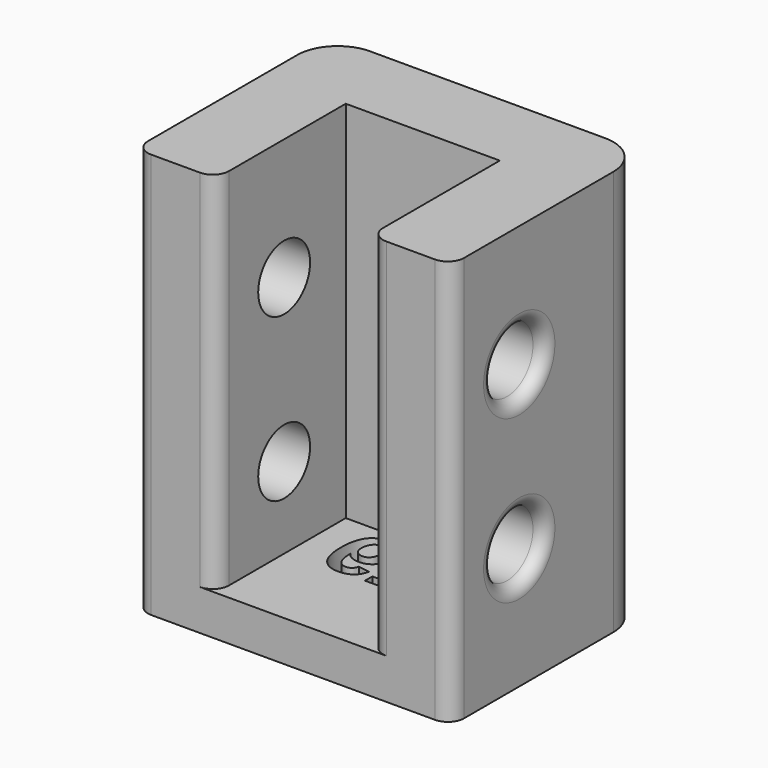
from build123d import *

# Parameters (mm, degrees)
F0_W         = 19
F0_H         = 20
F1_DEPTH     = 5
F2_DEPTH     = 50
F3_R         = 4
F4_DEPTH     = 40
F5_R         = 4
F6_DEPTH     = 10
F7_R         = 1.5
F8_TEXT_SIZE = 11.2298606202
F9_DEPTH     = 5
F10_R        = 5
F11_R        = 2


# Not quite as in the source:
# - Text() gives the source's letters only with a copy of the font that has no kerning and outlines rounded to 1/6400 em; it was checked with that copy


with BuildPart() as f1:
    # F0 (on Top) → F1 (new body)
    with BuildSketch(Plane.XY):
        Polygon((19.5, 15), (-19.5, 15), (-19.5, -15), (-9.5, -15), (-9.5, 5), (9.5, 5), (9.5, -15), (19.5, -15), align=None)
        with Locations((0, -5)):
            Rectangle(F0_W, F0_H)
    extrude(amount=F1_DEPTH)

    # F0 (on Top) → F2 (join)
    with BuildSketch(Plane.XY):
        Polygon((19.5, 15), (-19.5, 15), (-19.5, -15), (-9.5, -15), (-9.5, 5), (9.5, 5), (9.5, -15), (19.5, -15), align=None)
    extrude(amount=F2_DEPTH)

    # F3 (on face) → F4 (cut)
    with BuildSketch(Plane(origin=(-19.5, 0, 0), x_dir=(0, -1, 0), z_dir=(-1, 0, 0))):
        with Locations((4.5, 15)):
            Circle(F3_R)
        with Locations((4.5, 35)):
            Circle(F3_R)
    extrude(amount=-F4_DEPTH, mode=Mode.SUBTRACT)

    # F5 (on face) → F6 (cut)
    with BuildSketch(Plane(origin=(0, 15, 0), x_dir=(-1, 0, 0), z_dir=(0, 1, 0))):
        with Locations((0, 15)):
            Circle(F5_R)
        with Locations((0, 35)):
            Circle(F5_R)
    extrude(amount=-F6_DEPTH, mode=Mode.SUBTRACT)

    # F7
    f7_edges = [f1.edges().sort_by_distance(p)[0] for p in [
        (-19.5, -0.5, 15),
        (-19.5, -0.5, 35),
        (4, 15, 35),
        (4, 15, 15),
        (19.5, -0.5, 35),
        (19.5, -0.5, 15),
    ]]
    fillet(f7_edges, radius=F7_R)

    # F8 (on face) → F9 (cut)
    with BuildSketch(Plane(origin=(0, 0, 0), x_dir=(1, 0, 0), z_dir=(0, 0, -1))):
        with Locations(Location((6.0369274162, 4.0427498233), (0, 0, 180))):
            Text('19', F8_TEXT_SIZE, font='Arimo', font_style=FontStyle.BOLD, text_align=(TextAlign.LEFT, TextAlign.BOTTOM))
    extrude(amount=-F9_DEPTH, mode=Mode.SUBTRACT)

    # F10
    f10_edges = [f1.edges().sort_by_distance(p)[0] for p in [
        (19.5, 15, 25),
        (-19.5, 15, 25),
    ]]
    fillet(f10_edges, radius=F10_R)

    # F11
    f11_edges = [f1.edges().sort_by_distance(p)[0] for p in [
        (-9.5, -15, 27.5),
        (9.5, -15, 27.5),
        (19.5, -15, 25),
        (-19.5, -15, 25),
    ]]
    fillet(f11_edges, radius=F11_R)


solid = f1.part
